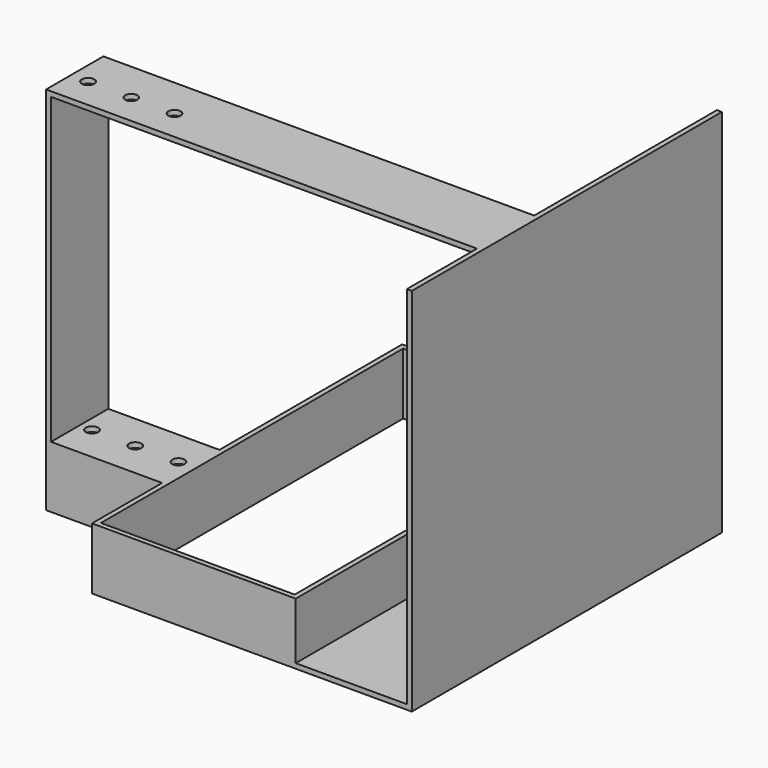
from build123d import *

# Parameters (mm, degrees)
F0_W          = 165
F0_H          = 314
F0_W_2        = 157
F0_H_2        = 306
F1_DEPTH      = 50
F3_DEPTH      = 90
F4_R          = 5
F5_DEPTH      = 14
F5_DEPTH_BACK = 70
F6_DEPTH      = 50
F7_W          = 4
F7_H          = 58
F8_DEPTH      = 300
F9_W          = 58
F9_H          = 4
F10_DEPTH     = 345
F11_W         = 314
F11_H         = 4
F12_DEPTH     = 90
F13_W         = 4
F13_H         = 314
F14_DEPTH     = 300
F15_R         = 5
F16_DEPTH     = 29


# Not quite as in the source:
# - a feature names something its author has since deleted; it is built from what else it names


with BuildPart() as f1:
    # F0 (on Top) → F1 (new body)
    with BuildSketch(Plane.XY):
        with Locations((0, -8.0325696617)):
            Rectangle(F0_W, F0_H)
        with Locations((0, -8.0325696617)):
            Rectangle(F0_W_2, F0_H_2, mode=Mode.SUBTRACT)
    extrude(amount=F1_DEPTH)

    # F2 (on face) → F3 (join)
    with BuildSketch(Plane(origin=(-82.5, 0, 0), x_dir=(0, -1, 0), z_dir=(-1, 0, 0))):
        Polygon((36.0325696617, 0), (65.0325696617, 0), (65.0325696617, 4), (40.0325696617, 4), (40.0325696617, 46), (65.0325696617, 46), (65.0325696617, 50), (36.0325696617, 50), align=None)
        Polygon((65.0325696617, 4), (65.0325696617, 0), (94.0325696617, 0), (94.0325696617, 50), (65.0325696617, 50), (65.0325696617, 46), (90.0325696617, 46), (90.0325696617, 4), align=None)
    extrude(amount=F3_DEPTH)

    # F4 (on face) → F5 (cut, two sides)
    with BuildSketch(Plane.XY.offset(4)) as f5_sk:
        with Locations((-92.5, -65.0325696617)):
            Circle(F4_R)
        with Locations((-162.5, -65.0325696617)):
            Circle(F4_R)
    extrude(amount=-F5_DEPTH, mode=Mode.SUBTRACT)
    extrude(f5_sk.sketch, amount=F5_DEPTH_BACK, mode=Mode.SUBTRACT)

    # F4 (on face) → F6 (cut)
    with BuildSketch(Plane.XY.offset(4)):
        with Locations((-127.5, -65.0325696617)):
            Circle(F4_R)
    extrude(amount=F6_DEPTH, mode=Mode.SUBTRACT)

    # F7 (on face) → F8 (join)
    with BuildSketch(Plane(origin=(0, 0, 0), x_dir=(1, 0, 0), z_dir=(0, 0, -1))):
        with Locations((-174.5, 65.0325696617)):
            Rectangle(F7_W, F7_H)
    extrude(amount=-F8_DEPTH)

    # F9 (on face) → F10 (join)
    with BuildSketch(Plane.YZ.offset(-172.5)):
        with Locations((-65.0325696617, 298)):
            Rectangle(F9_W, F9_H)
    extrude(amount=F10_DEPTH)

    # F11 (on face) → F12 (join)
    with BuildSketch(Plane.YZ.offset(82.5)):
        with Locations((-8.0325696617, 2)):
            Rectangle(F11_W, F11_H)
    extrude(amount=F12_DEPTH)

    # F13 (on face) → F14 (join)
    with BuildSketch(Plane(origin=(0, 0, 0), x_dir=(1, 0, 0), z_dir=(0, 0, -1))):
        with Locations((174.5, 8.0325696617)):
            Rectangle(F13_W, F13_H)
    extrude(amount=-F14_DEPTH)

    # F15 (on face) → F16 (cut)
    with BuildSketch(Plane.XY.offset(300)):
        with Locations((-92.5, -69.0325696617)):
            Circle(F15_R)
        with Locations((-127.5, -69.0325696617)):
            Circle(F15_R)
        with Locations((-162.5, -69.0325696617)):
            Circle(F15_R)
    extrude(amount=-F16_DEPTH, mode=Mode.SUBTRACT)


solid = f1.part
